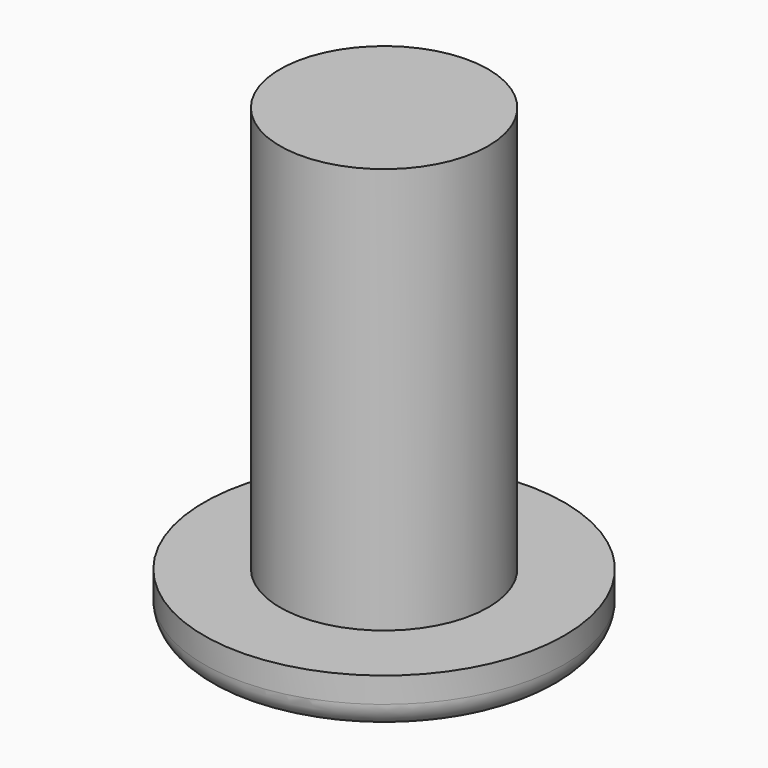
from build123d import *

# Parameters (mm, degrees)
F0_R     = 2.05
F1_DEPTH = 8
F2_R     = 3.55
F2_R_2   = 2.05
F3_DEPTH = 1
F4_R     = 0.5


with BuildPart() as f1:
    # F0 (on Top) → F1 (new body)
    with BuildSketch(Plane.XY):
        Circle(F0_R)
    extrude(amount=F1_DEPTH)

    # F2 (on face) → F3 (join)
    with BuildSketch(Plane(origin=(0, 0, 0), x_dir=(1, 0, 0), z_dir=(0, 0, -1))):
        Circle(F2_R)
        Circle(F2_R_2, mode=Mode.SUBTRACT)
        Circle(F2_R_2)
    extrude(amount=F3_DEPTH)

    # F4
    f4_edges = [f1.edges().sort_by_distance(p)[0] for p in [
        (-3.55, 0, -1),
    ]]
    fillet(f4_edges, radius=F4_R)


solid = f1.part
